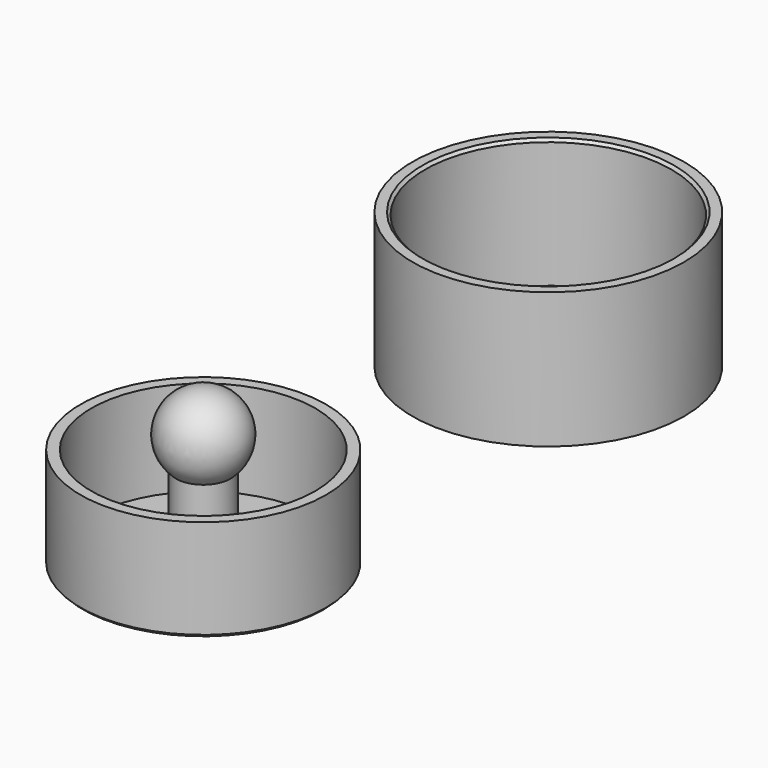
from build123d import *

# Parameters (mm, degrees)
F0_R         = 18.15
F0_R_2       = 2
F1_DEPTH     = 1
F0_R_3       = 16.5
F0_R_4       = 4
F0_R_5       = 20
F2_DEPTH     = 20
F0_R_6       = 18.075
F3_DEPTH     = 15
F4_DEPTH     = 17
F5_SIZE      = 0.4
F6_W         = 0.6
F6_H         = 13
F6_W_2       = 13
F6_H_2       = 0.6
F6_TEXT_SIZE = 5.5555555556
F7_DEPTH     = 0.2
F8_W         = 1.1
F8_H         = 9.9801421165
F8_W_2       = 10.9774479643
F8_H_2       = 1.0481402278
F8_TEXT_SIZE = 5.7179987005
F9_DEPTH     = 0.2
F10_SIZE     = 0.4


# Not quite as in the source:
# - Text() gives the source's letters only with a copy of the font that has no kerning and outlines rounded to 1/6400 em; it was checked with that copy


with BuildPart() as f1:
    # F0 (on Top) → F1 (new body)
    with BuildSketch(Plane.XY):
        Circle(F0_R)
        Circle(F0_R_2, mode=Mode.SUBTRACT)
    extrude(amount=F1_DEPTH)

    # F0 (on Top) → F2 (join)
    with BuildSketch(Plane.XY):
        Circle(F0_R_5)
        Circle(F0_R, mode=Mode.SUBTRACT)
    extrude(amount=F2_DEPTH)

    # F5
    f5_edges = [f1.edges().sort_by_distance(p)[0] for p in [
        (-18.15, 0, 20),
    ]]
    chamfer(f5_edges, length=F5_SIZE)

    # F6 (on face) → F7 (join)
    with BuildSketch(Plane.XY.offset(1)):
        with Locations((0.3, 10.5)):
            Rectangle(F6_W, F6_H)
        with Locations((10.5, -0.3)):
            Rectangle(F6_W_2, F6_H_2)
        with Locations((11.9159572819, 1.6112038437)):
            Text('X', F6_TEXT_SIZE, font='Open Sans', font_style=FontStyle.BOLD, text_align=(TextAlign.LEFT, TextAlign.BOTTOM))
        with Locations((1.9039693579, 11.2683388442)):
            Text('Y', F6_TEXT_SIZE, font='Open Sans', font_style=FontStyle.BOLD, text_align=(TextAlign.LEFT, TextAlign.BOTTOM))
    extrude(amount=F7_DEPTH)


with BuildPart() as f1b:
    # F0 (on Top) → F1, piece 2 (new body)
    with BuildSketch(Plane.XY):
        with Locations((0, -63.4981170297)):
            Circle(F0_R_3)
        with Locations((0, -63.4981170297)):
            Circle(F0_R_4, mode=Mode.SUBTRACT)
    extrude(amount=F1_DEPTH)

    # F0 (on Top) → F3 (join)
    with BuildSketch(Plane.XY):
        with Locations((0, -63.4981170297)):
            Circle(F0_R_6)
        with Locations((0, -63.4981170297)):
            Circle(F0_R_3, mode=Mode.SUBTRACT)
    extrude(amount=F3_DEPTH)

    # F0 (on Top) → F4 (join)
    with BuildSketch(Plane.XY):
        with Locations((0, -63.4981170297)):
            Circle(F0_R_4)
    extrude(amount=F4_DEPTH)

    # F8 (on face) → F9 (join)
    with BuildSketch(Plane.XY.offset(1)):
        with Locations((0.55, -53.4064285457)):
            Rectangle(F8_W, F8_H)
        with Locations((10.3780510835, -63.6624507606)):
            Rectangle(F8_W_2, F8_H_2)
        with Locations((-8.0537942704, -74.9272696069)):
            Text('0.15', F8_TEXT_SIZE, font='Open Sans', text_align=(TextAlign.LEFT, TextAlign.BOTTOM))
    extrude(amount=F9_DEPTH)

    # F10
    f10_edges = [f1b.edges().sort_by_distance(p)[0] for p in [
        (-18.075, -63.498117, 0),
    ]]
    chamfer(f10_edges, length=F10_SIZE)

    # F11 (on face) → F12 (revolve)
    with BuildSketch(Plane.XY.offset(17)):
        with BuildLine():
            Line((-4, -63.4981170297), (-6, -63.4981170297))
            ThreePointArc((-6, -63.4981170297), (0, -69.4981170297), (6, -63.4981170297))
            Line((6, -63.4981170297), (4, -63.4981170297))
            ThreePointArc((4, -63.4981170297), (0, -67.4981170297), (-4, -63.4981170297))
        make_face()
        with BuildLine():
            Line((4, -63.4981170297), (-4, -63.4981170297))
            ThreePointArc((-4, -63.4981170297), (0, -67.4981170297), (4, -63.4981170297))
        make_face()
    revolve(axis=Axis((-14.8261445314, -63.4981170297, 17), (1, 0, 0)))


solid = Compound([f1.part, f1b.part])
